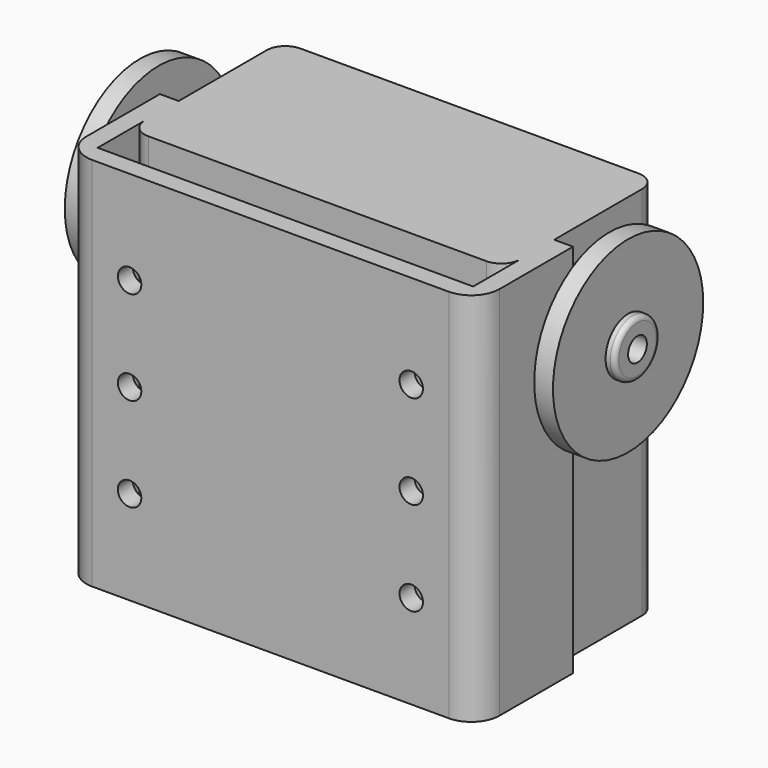
from build123d import *

# Parameters (mm, degrees)
F0_W            = 40
F0_H            = 20.25
F1_DEPTH        = 40
F2_R            = 2
F3_R            = 6.5
F4_DEPTH        = 2
F5_SIZE2        = 0.29999
F5_SIZE         = 1.99999
F6_R            = 0.5
F7_R            = 3
F8_DEPTH        = 4
F9_R            = 0.5
F10_R           = 6.5
F11_DEPTH       = 2
F12_R           = 0.5
F13_R           = 3
F14_DEPTH       = 4
F15_R           = 0.5
F17_D           = 2.5
F17_DEPTH       = 3
F17_CBORE_D     = 2.5
F17_CBORE_DEPTH = 0
F17_TIP         = 0.7510757738
F19_D           = 2.5
F19_DEPTH       = 3
F19_CBORE_D     = 2.5
F19_CBORE_DEPTH = 0
F19_TIP         = 0.7510757738
F21_R           = 10
F21_R_2         = 1
F22_DEPTH       = 2
F24_R           = 10
F24_R_2         = 3
F25_DEPTH       = 2
F27_DEPTH       = 40
F28_R           = 3
F30_D           = 2.5
F30_DEPTH       = 3
F30_TIP         = 0.7510757738


# Not quite as in the source:
# - a fillet or chamfer is up to 0.001 mm smaller than in the source, because OpenCascade refuses the exact size


with BuildPart() as f1:
    # F0 (on Top) → F1 (new body)
    with BuildSketch(Plane.XY):
        Rectangle(F0_W, F0_H)
    extrude(amount=F1_DEPTH)

    # F2
    f2_edges = [f1.edges().sort_by_distance(p)[0] for p in [
        (-20, 10.125, 20),
        (-20, -10.125, 20),
        (20, 10.125, 20),
        (20, -10.125, 20),
    ]]
    fillet(f2_edges, radius=F2_R)

    # F3 (on face) → F4 (join)
    with BuildSketch(Plane(origin=(-20, 0, 0), x_dir=(0, -1, 0), z_dir=(-1, 0, 0))):
        with Locations((0, 30.225)):
            Circle(F3_R)
    extrude(amount=F4_DEPTH)

    # F5 (size 2 and 0.3 in the source; OpenCascade refuses exactly that, so slightly less here)
    f5_edges = [f1.edges().sort_by_distance(p)[0] for p in [
        (-22, 6.5, 30.225),
    ]]
    chamfer(f5_edges, length=F5_SIZE, length2=F5_SIZE2)

    # F6
    f6_edges = [f1.edges().sort_by_distance(p)[0] for p in [
        (-22, 6.20001, 30.225),
    ]]
    fillet(f6_edges, radius=F6_R)

    # F7 (on face) → F8 (join)
    with BuildSketch(Plane(origin=(-22, 0, 0), x_dir=(0, -1, 0), z_dir=(-1, 0, 0))):
        with Locations((0, 30.225)):
            Circle(F7_R)
    extrude(amount=F8_DEPTH)

    # F9
    f9_edges = [f1.edges().sort_by_distance(p)[0] for p in [
        (-26, 3, 30.225),
    ]]
    fillet(f9_edges, radius=F9_R)

    # F10 (on face) → F11 (join)
    with BuildSketch(Plane.YZ.offset(20)):
        with Locations((0, 30.225)):
            Circle(F10_R)
    extrude(amount=F11_DEPTH)

    # F12
    f12_edges = [f1.edges().sort_by_distance(p)[0] for p in [
        (22, -6.5, 30.225),
    ]]
    fillet(f12_edges, radius=F12_R)

    # F13 (on face) → F14 (join)
    with BuildSketch(Plane.YZ.offset(22)):
        with Locations((0, 30.225)):
            Circle(F13_R)
    extrude(amount=F14_DEPTH)

    # F15
    f15_edges = [f1.edges().sort_by_distance(p)[0] for p in [
        (26, -3, 30.225),
    ]]
    fillet(f15_edges, radius=F15_R)

    # F17
    with Locations(Plane(origin=(-26, 0, 0), x_dir=(0, -1, 0), z_dir=(-1, 0, 0))):
        with Locations((0, 30.225)):
            CounterBoreHole(F17_D / 2, F17_CBORE_D / 2, F17_CBORE_DEPTH, depth=F17_DEPTH)
            with Locations((0, 0, -(F17_DEPTH + F17_TIP / 2))):  # 118° drill point
                Cone(0, F17_D / 2, F17_TIP, mode=Mode.SUBTRACT)

    # F19
    with Locations(Plane.YZ.offset(26)):
        with Locations((0, 30.225)):
            CounterBoreHole(F19_D / 2, F19_CBORE_D / 2, F19_CBORE_DEPTH, depth=F19_DEPTH)
            with Locations((0, 0, -(F19_DEPTH + F19_TIP / 2))):  # 118° drill point
                Cone(0, F19_D / 2, F19_TIP, mode=Mode.SUBTRACT)

    # F21 (on offset) → F22 (join)
    with BuildSketch(Plane(origin=(-27, 0, 0), x_dir=(0, -1, 0), z_dir=(-1, 0, 0))):
        with Locations((0, 30.225)):
            Circle(F21_R)
        with Locations((0, 30.225)):
            Circle(F21_R_2, mode=Mode.SUBTRACT)
    extrude(amount=-F22_DEPTH)

    # F24 (on offset) → F25 (join)
    with BuildSketch(Plane.YZ.offset(25)):
        with Locations((0, 30.225)):
            Circle(F24_R)
        with Locations((0, 30.225)):
            Circle(F24_R_2, mode=Mode.SUBTRACT)
    extrude(amount=-F25_DEPTH)

    # F26 (on Top) → F27 (join)
    with BuildSketch(Plane.XY):
        Polygon((22, -16.375), (22, -3.5868030973), (20, -3.5868030973), (20, -14.375), (-20, -14.375), (-20, -3.5868030973), (-22, -3.5868030973), (-22, -16.375), align=None)
    extrude(amount=F27_DEPTH)

    # F28
    f28_edges = [f1.edges().sort_by_distance(p)[0] for p in [
        (22, -16.375, 20),
        (-22, -16.375, 20),
    ]]
    fillet(f28_edges, radius=F28_R)

    # F30
    with Locations(Plane.XZ.offset(16.375)):
        with Locations((-15, 30), (15, 30), (15, 20), (-15, 20), (-15, 10), (15, 10)):
            Hole(F30_D / 2, depth=F30_DEPTH)
            with Locations((0, 0, -(F30_DEPTH + F30_TIP / 2))):  # 118° drill point
                Cone(0, F30_D / 2, F30_TIP, mode=Mode.SUBTRACT)


solid = f1.part
